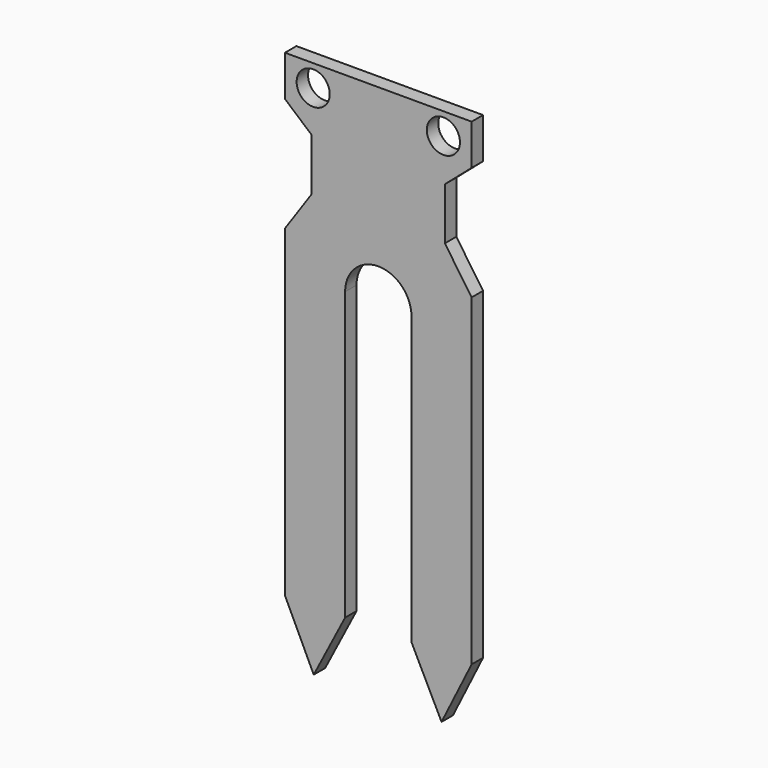
from build123d import *

# Parameters (mm, degrees)
F0_R     = 1.76
F1_DEPTH = 1.52


# Not quite as in the source:
# - a feature of the source that left no trace in its solid (it failed there, or was rolled back) is left out


with BuildPart() as f1:
    # F0 (on Front) → F1 (new body)
    with BuildSketch(Plane.XZ):
        Polygon((-13.44, 42.2827300502), (-19.83, 42.2827300502), (-19.83, 41.2284731865), (-19.83, 38.147136569), (-19.83, 37.9599481821), (-16.99, 35.5119891465), (-16.99, 29.9802143127), (-19.83, 25.8499481821), (-19.83, 25.4327300502), (-19.83, 22.0077300502), (-13.44, 22.0077300502), align=None)
        with Locations((-16.83, 39.9527300502)):
            Circle(F0_R, mode=Mode.SUBTRACT)
        with BuildLine():
            Line((-9.915, 42.2827300502), (-13.44, 42.2827300502))
            Line((-13.44, 42.2827300502), (-13.44, 22.0077300502))
            ThreePointArc((-13.44, 22.0077300502), (-12.4075514037, 24.5002814538), (-9.915, 25.5327300502))
            Line((-9.915, 25.5327300502), (-9.915, 42.2827300502))
        make_face()
        Polygon((-13.44, 22.0005065203), (-13.44, 22.0077300502), (-19.83, 22.0077300502), (-19.83, -8.4672699498), (-13.44, -8.4672699498), align=None)
        with BuildLine():
            Line((-6.39, 42.2827300502), (-9.915, 42.2827300502))
            Line((-9.915, 42.2827300502), (-9.915, 25.5327300502))
            ThreePointArc((-9.915, 25.5327300502), (-7.4224485963, 24.5002814538), (-6.39, 22.0077300502))
            Line((-6.39, 22.0077300502), (-6.39, 23.0757091194))
            Line((-6.39, 23.0757091194), (-6.39, 42.2827300502))
        make_face()
        Polygon((0, 42.2827300502), (-6.39, 42.2827300502), (-6.39, 23.0757091194), (-6.39, 22.0077300502), (-6.39, -8.4672699498), (0, -8.4672699498), (0, 25.4327300502), (0, 25.8499481821), (-2.84, 29.9802143127), (-2.84, 35.5119891465), (0, 37.9599481821), (0, 41.2284731865), align=None)
        with Locations((-3, 39.9527300502)):
            Circle(F0_R, mode=Mode.SUBTRACT)
        Polygon((-16.7724229395, -14.8872699498), (-13.44, -8.4672699498), (-19.83, -8.4672699498), align=None)
        Polygon((0, -8.4672699498), (-6.39, -8.4672699498), (-3.195, -14.8872699498), align=None)
    extrude(amount=F1_DEPTH)


solid = f1.part
